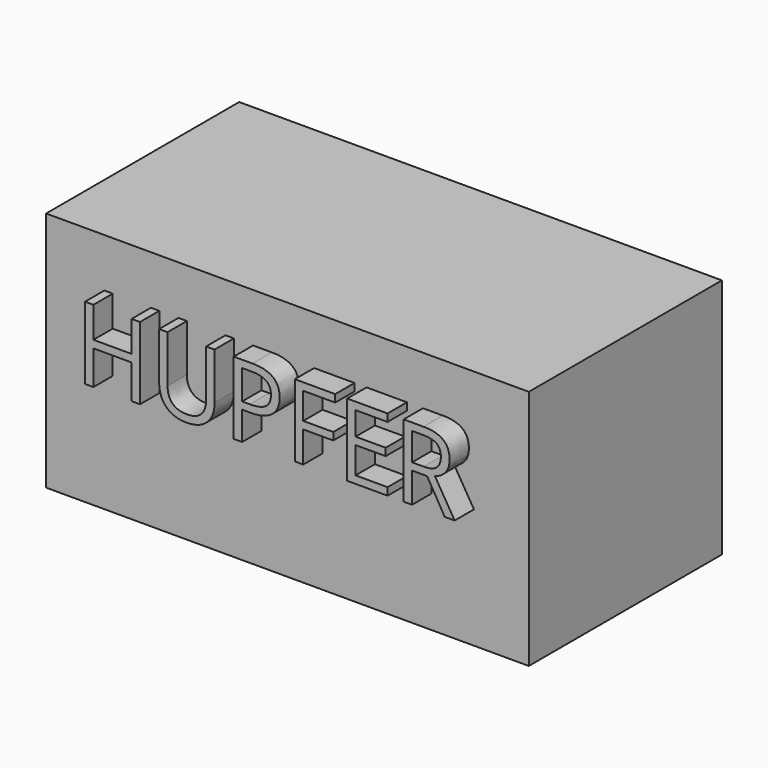
from build123d import *

# Parameters (mm, degrees)
F0_W         = 25.4
F0_H         = 12.7
F1_DEPTH     = 12.7
F2_TEXT_SIZE = 5.3390261926
F3_DEPTH     = 1.27


# Not quite as in the source:
# - Text() gives the source's letters only with a copy of the font that has no kerning and outlines rounded to 1/6400 em; it was checked with that copy


with BuildPart() as f1:
    # F0 (on Front) → F1 (new body)
    with BuildSketch(Plane.XZ):
        with Locations((3.7678005174, 2.9806787502)):
            Rectangle(F0_W, F0_H)
    extrude(amount=F1_DEPTH)

    # F2 (on face) → F3 (join)
    with BuildSketch(Plane.XZ.offset(12.7)):
        with Locations((-6.3921994826, 2.9465798915)):
            Text('HUPFER', F2_TEXT_SIZE, font='Open Sans', text_align=(TextAlign.LEFT, TextAlign.BOTTOM))
    extrude(amount=F3_DEPTH)


solid = f1.part
